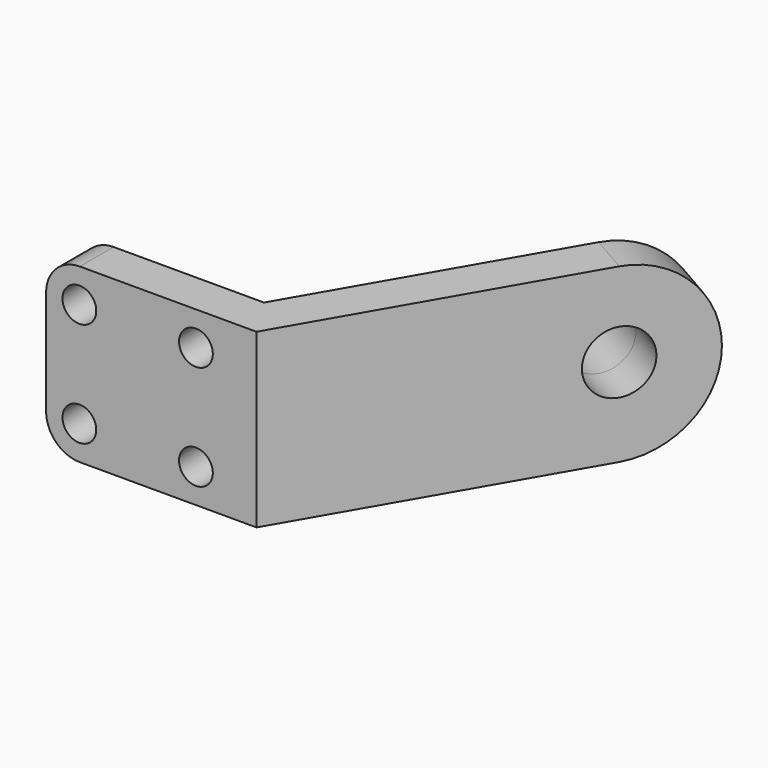
from build123d import *

# Parameters (mm, degrees)
F1_DEPTH  = 102
F2_R      = 27
F2_R_2    = 18.5
F3_DEPTH  = 30
F4_R      = 10
F5_DEPTH  = 50
F6_R      = 50.99999
F9_DEPTH  = 10
F10_R     = 18.5
F11_DEPTH = 30
F12_R     = 20


# Not quite as in the source:
# - a fillet or chamfer is up to 0.001 mm smaller than in the source, because OpenCascade refuses the exact size


with BuildPart() as f1:
    # F0 (on Top) → F1 (new body)
    with BuildSketch(Plane.XY):
        Polygon((-151.6251202653, -131.7925444834), (-151.6251202653, -156.7925444834), (-27.0366629971, -156.7925444834), (88.4633370029, 43.2593237909), (65.9466765045, 56.2593237909), (-42.6251202653, -131.7925444834), align=None)
    extrude(amount=F1_DEPTH)

    # F2 (on face) → F3 (join)
    with BuildSketch(Plane(origin=(25.099005577, -14.4909176263, 0), x_dir=(-0.5, -0.8660254038, 0), z_dir=(-0.8660254038, 0.5, 0))):
        with Locations((-30.6953418548, 52.0583279431)):
            Circle(F2_R)
        with Locations((-30.6953418548, 52.0583279431)):
            Circle(F2_R_2, mode=Mode.SUBTRACT)
    extrude(amount=F3_DEPTH)

    # F4 (on face) → F5 (cut)
    with BuildSketch(Plane(origin=(0, -131.7925444834, 0), x_dir=(-1, 0, 0), z_dir=(0, 1, 0))):
        with Locations((62.9175528884, 82)):
            Circle(F4_R)
        with Locations((131.9175528884, 82)):
            Circle(F4_R)
        with Locations((131.9175528884, 20)):
            Circle(F4_R)
        with Locations((62.9175528884, 20)):
            Circle(F4_R)
    extrude(amount=-F5_DEPTH, mode=Mode.SUBTRACT)

    # F6 (radius 51 in the source; OpenCascade refuses exactly that, so slightly less here)
    f6_edges = [f1.edges().sort_by_distance(p)[0] for p in [
        (77.205007, 49.759324, 102),
        (77.205007, 49.759324, 0),
    ]]
    fillet(f6_edges, radius=F6_R)

    # F8 (on offset) → F9 (join, symmetric)
    with BuildSketch(Plane(origin=(0, 0, 51), x_dir=(1, 0, 0), z_dir=(0, 0, -1))):
        Polygon((-42.6251202653, 131.7925444834), (-151.6251202653, 131.7925444834), (-4.3144722301, 66.1549466668), align=None)
    extrude(amount=F9_DEPTH, both=True)

    # F10 (on face) → F11 (cut)
    with BuildSketch(Plane(origin=(25.099005577, -14.4909176263, 0), x_dir=(-0.5, -0.8660254038, 0), z_dir=(-0.8660254038, 0.5, 0))):
        with Locations((-30.6953418548, 52.0583279431)):
            Circle(F10_R)
    extrude(amount=-F11_DEPTH, mode=Mode.SUBTRACT)

    # F12
    f12_edges = [f1.edges().sort_by_distance(p)[0] for p in [
        (-151.62512, -144.292544, 102),
        (-151.62512, -144.292544, 0),
    ]]
    fillet(f12_edges, radius=F12_R)


solid = f1.part
